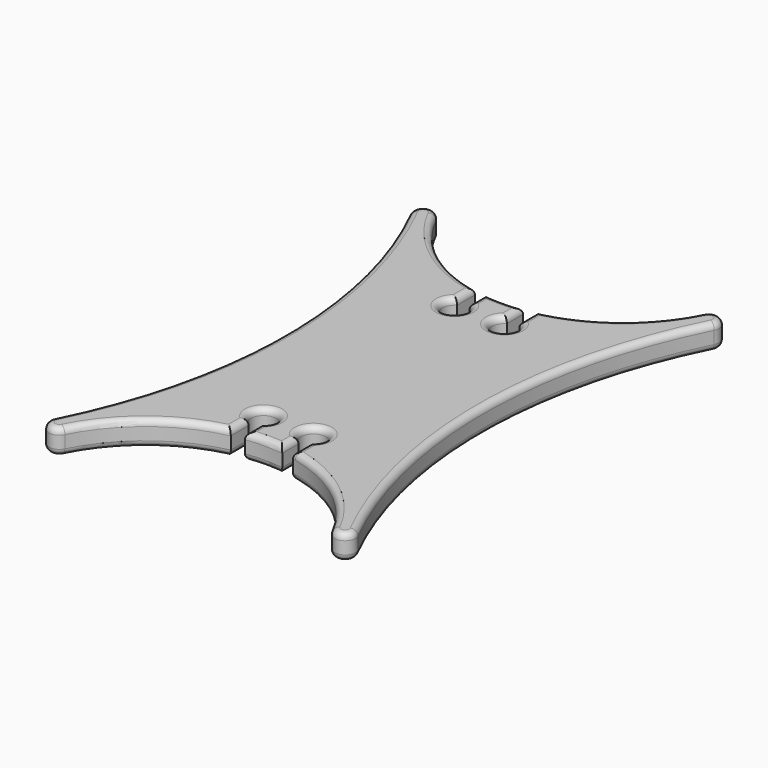
from build123d import *

# Parameters (mm, degrees)
F1_DEPTH     = 3.175
F2_T1_DEPTH  = 6.821932003
F2_T3_DEPTH  = 6.821932003
F2_T5_DEPTH  = 6.5533487431
F2_T7_DEPTH  = 6.5533487431
F2_T10_ANGLE = 359.64
F2_T12_ANGLE = 57.3793421658
F2_T14_ANGLE = 180
F2_T16_ANGLE = 53.1301023542
F2_T18_ANGLE = 180
F2_T20_ANGLE = 57.3793421658
F2_T22_ANGLE = 359.64
F2_T24_ANGLE = 26.298254359
F2_T26_ANGLE = 359.64
F2_T28_ANGLE = 57.3793421658
F2_T30_ANGLE = 180
F2_T32_ANGLE = 53.1301023542
F2_T34_ANGLE = 180
F2_T36_ANGLE = 57.3793421658
F2_T38_ANGLE = 359.64
F2_T40_ANGLE = 26.298254359
F2_T42_ANGLE = 359.64
F2_T44_ANGLE = 57.3793421658
F2_T46_ANGLE = 180
F2_T48_ANGLE = 53.1301023542
F2_T50_ANGLE = 180
F2_T52_ANGLE = 57.3793421658
F2_T54_ANGLE = 359.64
F2_T56_ANGLE = 26.298254359
F2_T58_ANGLE = 359.64
F2_T60_ANGLE = 57.3793421658
F2_T62_ANGLE = 180
F2_T64_ANGLE = 53.1301023542
F2_T66_ANGLE = 180
F2_T68_ANGLE = 57.3793421658
F2_T70_ANGLE = 359.64
F2_T72_ANGLE = 26.298254359


# Not quite as in the source:
# - a fillet or chamfer that OpenCascade refuses, or shapes differently, is made with other operations: its cross-section is extruded or revolved along the edge and cut away or added


with BuildPart() as f1:
    # F0 (on Top) → F1 (new body)
    with BuildSketch(Plane.XY):
        with BuildLine():
            ThreePointArc((-3.96875, 19.4679973315), (-11.6574343411, 23.0332576652), (-17.0388379885, 29.5805810057))
            ThreePointArc((-17.0388379885, 29.5805810057), (-18.8126145258, 30.1718398515), (-19.4038733715, 28.3980633142))
            ThreePointArc((-19.4038733715, 28.3980633142), (-12.7, 0), (-19.4038733715, -28.3980633142))
            ThreePointArc((-19.4038733715, -28.3980633142), (-18.8126145258, -30.1718398515), (-17.0388379885, -29.5805810057))
            ThreePointArc((-17.0388379885, -29.5805810057), (-11.6574343411, -23.0332576652), (-3.96875, -19.4679973315))
            Line((-3.96875, -19.4679973315), (-3.96875, -16.6148153285))
            ThreePointArc((-3.96875, -16.6148153285), (-3.175, -13.6525), (-2.38125, -16.6148153285))
            Line((-2.38125, -16.6148153285), (-2.38125, -19.1994140716))
            ThreePointArc((-2.38125, -19.1994140716), (0, -19.05), (2.38125, -19.1994140716))
            Line((2.38125, -19.1994140716), (2.38125, -16.6148153285))
            ThreePointArc((2.38125, -16.6148153285), (3.175, -13.6525), (3.96875, -16.6148153285))
            Line((3.96875, -16.6148153285), (3.96875, -19.4679973315))
            ThreePointArc((3.96875, -19.4679973315), (11.6574343411, -23.0332576652), (17.0388379885, -29.5805810057))
            ThreePointArc((17.0388379885, -29.5805810057), (18.8126145258, -30.1718398515), (19.4038733715, -28.3980633142))
            ThreePointArc((19.4038733715, -28.3980633142), (12.7, 0), (19.4038733715, 28.3980633142))
            ThreePointArc((19.4038733715, 28.3980633142), (18.8126145258, 30.1718398515), (17.0388379885, 29.5805810057))
            ThreePointArc((17.0388379885, 29.5805810057), (11.6574343411, 23.0332576652), (3.96875, 19.4679973315))
            Line((3.96875, 19.4679973315), (3.96875, 16.6148153285))
            ThreePointArc((3.96875, 16.6148153285), (3.175, 13.6525), (2.38125, 16.6148153285))
            Line((2.38125, 16.6148153285), (2.38125, 19.1994140716))
            ThreePointArc((2.38125, 19.1994140716), (0, 19.05), (-2.38125, 19.1994140716))
            Line((-2.38125, 19.1994140716), (-2.38125, 16.6148153285))
            ThreePointArc((-2.38125, 16.6148153285), (-3.175, 13.6525), (-3.96875, 16.6148153285))
            Line((-3.96875, 16.6148153285), (-3.96875, 19.4679973315))
        make_face()
    extrude(amount=F1_DEPTH)

    # F2: fillet of radius 0.79375 on 48 edges, made by hand

    # F2_s2 → F2_t1 (cut)
    with BuildSketch(Plane.XZ.offset(-21.4523723315)):
        with BuildLine():
            ThreePointArc((-3.96875, 2.38125), (-4.2012339924, 2.9425160076), (-4.7625, 3.175))
            Line((-4.7625, 3.175), (-3.96875, 3.175))
            Line((-3.96875, 3.175), (-3.96875, 2.38125))
        make_face()
        with BuildLine():
            ThreePointArc((3.96875, 2.38125), (4.2012339924, 2.9425160076), (4.7625, 3.175))
            Line((4.7625, 3.175), (3.96875, 3.175))
            Line((3.96875, 3.175), (3.96875, 2.38125))
        make_face()
        with BuildLine():
            ThreePointArc((-3.96875, 0.79375), (-4.2012339924, 0.2324839924), (-4.7625, 0))
            Line((-4.7625, 0), (-3.96875, 0))
            Line((-3.96875, 0), (-3.96875, 0.79375))
        make_face()
        with BuildLine():
            ThreePointArc((3.96875, 0.79375), (4.2012339924, 0.2324839924), (4.7625, 0))
            Line((4.7625, 0), (3.96875, 0))
            Line((3.96875, 0), (3.96875, 0.79375))
        make_face()
    extrude(amount=F2_T1_DEPTH, mode=Mode.SUBTRACT)

    # F2_s4 → F2_t3 (cut)
    with BuildSketch(Plane.XZ.offset(14.6304403285)):
        with BuildLine():
            ThreePointArc((-3.96875, 2.38125), (-4.2012339924, 2.9425160076), (-4.7625, 3.175))
            Line((-4.7625, 3.175), (-3.96875, 3.175))
            Line((-3.96875, 3.175), (-3.96875, 2.38125))
        make_face()
        with BuildLine():
            ThreePointArc((3.96875, 2.38125), (4.2012339924, 2.9425160076), (4.7625, 3.175))
            Line((4.7625, 3.175), (3.96875, 3.175))
            Line((3.96875, 3.175), (3.96875, 2.38125))
        make_face()
        with BuildLine():
            ThreePointArc((-3.96875, 0.79375), (-4.2012339924, 0.2324839924), (-4.7625, 0))
            Line((-4.7625, 0), (-3.96875, 0))
            Line((-3.96875, 0), (-3.96875, 0.79375))
        make_face()
        with BuildLine():
            ThreePointArc((3.96875, 0.79375), (4.2012339924, 0.2324839924), (4.7625, 0))
            Line((4.7625, 0), (3.96875, 0))
            Line((3.96875, 0), (3.96875, 0.79375))
        make_face()
    extrude(amount=F2_T3_DEPTH, mode=Mode.SUBTRACT)

    # F2_s6 → F2_t5 (cut)
    with BuildSketch(Plane.XZ.offset(14.6304403285)):
        with BuildLine():
            ThreePointArc((-2.38125, 2.38125), (-2.1487660076, 2.9425160076), (-1.5875, 3.175))
            Line((-1.5875, 3.175), (-2.38125, 3.175))
            Line((-2.38125, 3.175), (-2.38125, 2.38125))
        make_face()
        with BuildLine():
            ThreePointArc((2.38125, 2.38125), (2.1487660076, 2.9425160076), (1.5875, 3.175))
            Line((1.5875, 3.175), (2.38125, 3.175))
            Line((2.38125, 3.175), (2.38125, 2.38125))
        make_face()
        with BuildLine():
            ThreePointArc((-2.38125, 0.79375), (-2.1487660076, 0.2324839924), (-1.5875, 0))
            Line((-1.5875, 0), (-2.38125, 0))
            Line((-2.38125, 0), (-2.38125, 0.79375))
        make_face()
        with BuildLine():
            ThreePointArc((2.38125, 0.79375), (2.1487660076, 0.2324839924), (1.5875, 0))
            Line((1.5875, 0), (2.38125, 0))
            Line((2.38125, 0), (2.38125, 0.79375))
        make_face()
    extrude(amount=F2_T5_DEPTH, mode=Mode.SUBTRACT)

    # F2_s8 → F2_t7 (cut)
    with BuildSketch(Plane.XZ.offset(-21.1837890716)):
        with BuildLine():
            ThreePointArc((2.38125, 2.38125), (2.1487660076, 2.9425160076), (1.5875, 3.175))
            Line((1.5875, 3.175), (2.38125, 3.175))
            Line((2.38125, 3.175), (2.38125, 2.38125))
        make_face()
        with BuildLine():
            ThreePointArc((-2.38125, 2.38125), (-2.1487660076, 2.9425160076), (-1.5875, 3.175))
            Line((-1.5875, 3.175), (-2.38125, 3.175))
            Line((-2.38125, 3.175), (-2.38125, 2.38125))
        make_face()
        with BuildLine():
            ThreePointArc((2.38125, 0.79375), (2.1487660076, 0.2324839924), (1.5875, 0))
            Line((1.5875, 0), (2.38125, 0))
            Line((2.38125, 0), (2.38125, 0.79375))
        make_face()
        with BuildLine():
            ThreePointArc((-2.38125, 0.79375), (-2.1487660076, 0.2324839924), (-1.5875, 0))
            Line((-1.5875, 0), (-2.38125, 0))
            Line((-2.38125, 0), (-2.38125, 0.79375))
        make_face()
    extrude(amount=F2_T7_DEPTH, mode=Mode.SUBTRACT)

    # F2_s9 → F2_t10 (revolve, cut)
    with BuildSketch(Plane(origin=(-3.2228462211, 0.0101249033, 0), x_dir=(0, 0, 1), z_dir=(-0.9999950652, 0.0031415875, 0))):
        with BuildLine():
            ThreePointArc((2.38125, 16.8174502534), (2.9425160076, 17.0499342458), (3.175, 17.6112002534))
            Line((3.175, 17.6112002534), (3.175, 16.8174502534))
            Line((3.175, 16.8174502534), (2.38125, 16.8174502534))
        make_face()
    revolve(axis=Axis((-3.175, 15.24, 3.175), (0, 0, -1)), revolution_arc=F2_T10_ANGLE, mode=Mode.SUBTRACT)

    # F2_s11 → F2_t12 (revolve, cut)
    with BuildSketch(Plane(origin=(-3.9968789782, 0.4240112092, 0), x_dir=(0, 0, 1), z_dir=(0.9944199801, -0.1054936165, 0))):
        with BuildLine():
            ThreePointArc((2.38125, -18.8374012427), (2.9425160076, -18.6049172503), (3.175, -18.0436512427))
            Line((3.175, -18.0436512427), (3.175, -18.8374012427))
            Line((3.175, -18.8374012427), (2.38125, -18.8374012427))
        make_face()
    revolve(axis=Axis((0, 38.1, 3.175), (0, 0, -1)), revolution_arc=F2_T12_ANGLE, mode=Mode.SUBTRACT)

    # F2_s13 → F2_t14 (revolve, cut)
    with BuildSketch(Plane(origin=(-15.24, 30.48, 0), x_dir=(0, 0, 1), z_dir=(0.4472135955, -0.894427191, 0))):
        with BuildLine():
            ThreePointArc((2.38125, 2.0111620115), (2.9425160076, 2.2436460039), (3.175, 2.8049120115))
            Line((3.175, 2.8049120115), (3.175, 2.0111620115))
            Line((3.175, 2.0111620115), (2.38125, 2.0111620115))
        make_face()
    revolve(axis=Axis((-18.22135568, 28.98932216, 3.175), (0, 0, 1)), revolution_arc=F2_T14_ANGLE, mode=Mode.SUBTRACT)

    # F2_s15 → F2_t16 (revolve, cut)
    with BuildSketch(Plane(origin=(-15.24, 30.48, 0), x_dir=(0, 0, 1), z_dir=(-0.4472135955, 0.894427191, 0))):
        with BuildLine():
            ThreePointArc((2.38125, -4.6553519542), (2.9425160076, -4.4228679618), (3.175, -3.8616019542))
            Line((3.175, -3.8616019542), (3.175, -4.6553519542))
            Line((3.175, -4.6553519542), (2.38125, -4.6553519542))
        make_face()
    revolve(axis=Axis((-76.2, 0, 3.175), (0, 0, -1)), revolution_arc=F2_T16_ANGLE, mode=Mode.SUBTRACT)

    # F2_s17 → F2_t18 (revolve, cut)
    with BuildSketch(Plane(origin=(-15.24, -30.48, 0), x_dir=(0, 0, 1), z_dir=(0.4472135955, 0.894427191, 0))):
        with BuildLine():
            ThreePointArc((2.38125, -4.6553519542), (2.9425160076, -4.4228679618), (3.175, -3.8616019542))
            Line((3.175, -3.8616019542), (3.175, -4.6553519542))
            Line((3.175, -4.6553519542), (2.38125, -4.6553519542))
        make_face()
    revolve(axis=Axis((-18.22135568, -28.98932216, 3.175), (0, 0, 1)), revolution_arc=F2_T18_ANGLE, mode=Mode.SUBTRACT)

    # F2_s19 → F2_t20 (revolve, cut)
    with BuildSketch(Plane(origin=(-15.24, -30.48, 0), x_dir=(0, 0, 1), z_dir=(-0.4472135955, -0.894427191, 0))):
        with BuildLine():
            ThreePointArc((2.38125, 2.0111620115), (2.9425160076, 2.2436460039), (3.175, 2.8049120115))
            Line((3.175, 2.8049120115), (3.175, 2.0111620115))
            Line((3.175, 2.0111620115), (2.38125, 2.0111620115))
        make_face()
    revolve(axis=Axis((0, -38.1, 3.175), (0, 0, -1)), revolution_arc=F2_T20_ANGLE, mode=Mode.SUBTRACT)

    # F2_s21 → F2_t22 (revolve, cut)
    with BuildSketch(Plane(origin=(-3.1270911071, 0.0098240788, 0), x_dir=(0, 0, 1), z_dir=(0.9999950652, -0.0031415875, 0))):
        with BuildLine():
            ThreePointArc((2.38125, 16.8373993339), (2.9425160076, 17.0698833264), (3.175, 17.6311493339))
            Line((3.175, 17.6311493339), (3.175, 16.8373993339))
            Line((3.175, 16.8373993339), (2.38125, 16.8373993339))
        make_face()
    revolve(axis=Axis((-3.175, -15.24, 3.175), (0, 0, -1)), revolution_arc=F2_T22_ANGLE, mode=Mode.SUBTRACT)

    # F2_s23 → F2_t24 (revolve, cut)
    with BuildSketch(Plane(origin=(-8.4399858607, -1.9716763507, 0), x_dir=(0, 0, 1), z_dir=(-0.9737812714, -0.2274863412, 0))):
        with BuildLine():
            ThreePointArc((2.38125, -18.0510664407), (2.9425160076, -17.8185824483), (3.175, -17.2573164407))
            Line((3.175, -17.2573164407), (3.175, -18.0510664407))
            Line((3.175, -18.0510664407), (2.38125, -18.0510664407))
        make_face()
    revolve(axis=Axis((0, -38.1, 3.175), (0, 0, -1)), revolution_arc=F2_T24_ANGLE, mode=Mode.SUBTRACT)

    # F2_s25 → F2_t26 (revolve, cut)
    with BuildSketch(Plane(origin=(3.2228462211, -0.0101249033, 0), x_dir=(0, 0, 1), z_dir=(0.9999950652, -0.0031415875, 0))):
        with BuildLine():
            ThreePointArc((2.38125, 16.8174502534), (2.9425160076, 17.0499342458), (3.175, 17.6112002534))
            Line((3.175, 17.6112002534), (3.175, 16.8174502534))
            Line((3.175, 16.8174502534), (2.38125, 16.8174502534))
        make_face()
    revolve(axis=Axis((3.175, -15.24, 3.175), (0, 0, -1)), revolution_arc=F2_T26_ANGLE, mode=Mode.SUBTRACT)

    # F2_s27 → F2_t28 (revolve, cut)
    with BuildSketch(Plane(origin=(3.9968789782, -0.4240112092, 0), x_dir=(0, 0, 1), z_dir=(-0.9944199801, 0.1054936165, 0))):
        with BuildLine():
            ThreePointArc((2.38125, -18.8374012427), (2.9425160076, -18.6049172503), (3.175, -18.0436512427))
            Line((3.175, -18.0436512427), (3.175, -18.8374012427))
            Line((3.175, -18.8374012427), (2.38125, -18.8374012427))
        make_face()
    revolve(axis=Axis((0, -38.1, 3.175), (0, 0, -1)), revolution_arc=F2_T28_ANGLE, mode=Mode.SUBTRACT)

    # F2_s29 → F2_t30 (revolve, cut)
    with BuildSketch(Plane(origin=(15.24, -30.48, 0), x_dir=(0, 0, 1), z_dir=(-0.4472135955, 0.894427191, 0))):
        with BuildLine():
            ThreePointArc((2.38125, 2.0111620115), (2.9425160076, 2.2436460039), (3.175, 2.8049120115))
            Line((3.175, 2.8049120115), (3.175, 2.0111620115))
            Line((3.175, 2.0111620115), (2.38125, 2.0111620115))
        make_face()
    revolve(axis=Axis((18.22135568, -28.98932216, 3.175), (0, 0, 1)), revolution_arc=F2_T30_ANGLE, mode=Mode.SUBTRACT)

    # F2_s31 → F2_t32 (revolve, cut)
    with BuildSketch(Plane(origin=(15.24, -30.48, 0), x_dir=(0, 0, 1), z_dir=(0.4472135955, -0.894427191, 0))):
        with BuildLine():
            ThreePointArc((2.38125, -4.6553519542), (2.9425160076, -4.4228679618), (3.175, -3.8616019542))
            Line((3.175, -3.8616019542), (3.175, -4.6553519542))
            Line((3.175, -4.6553519542), (2.38125, -4.6553519542))
        make_face()
    revolve(axis=Axis((76.2, 0, 3.175), (0, 0, -1)), revolution_arc=F2_T32_ANGLE, mode=Mode.SUBTRACT)

    # F2_s33 → F2_t34 (revolve, cut)
    with BuildSketch(Plane(origin=(15.24, 30.48, 0), x_dir=(0, 0, 1), z_dir=(-0.4472135955, -0.894427191, 0))):
        with BuildLine():
            ThreePointArc((2.38125, -4.6553519542), (2.9425160076, -4.4228679618), (3.175, -3.8616019542))
            Line((3.175, -3.8616019542), (3.175, -4.6553519542))
            Line((3.175, -4.6553519542), (2.38125, -4.6553519542))
        make_face()
    revolve(axis=Axis((18.22135568, 28.98932216, 3.175), (0, 0, 1)), revolution_arc=F2_T34_ANGLE, mode=Mode.SUBTRACT)

    # F2_s35 → F2_t36 (revolve, cut)
    with BuildSketch(Plane(origin=(15.24, 30.48, 0), x_dir=(0, 0, 1), z_dir=(0.4472135955, 0.894427191, 0))):
        with BuildLine():
            ThreePointArc((2.38125, 2.0111620115), (2.9425160076, 2.2436460039), (3.175, 2.8049120115))
            Line((3.175, 2.8049120115), (3.175, 2.0111620115))
            Line((3.175, 2.0111620115), (2.38125, 2.0111620115))
        make_face()
    revolve(axis=Axis((0, 38.1, 3.175), (0, 0, -1)), revolution_arc=F2_T36_ANGLE, mode=Mode.SUBTRACT)

    # F2_s37 → F2_t38 (revolve, cut)
    with BuildSketch(Plane(origin=(3.1270911071, -0.0098240788, 0), x_dir=(0, 0, 1), z_dir=(-0.9999950652, 0.0031415875, 0))):
        with BuildLine():
            ThreePointArc((2.38125, 16.8373993339), (2.9425160076, 17.0698833264), (3.175, 17.6311493339))
            Line((3.175, 17.6311493339), (3.175, 16.8373993339))
            Line((3.175, 16.8373993339), (2.38125, 16.8373993339))
        make_face()
    revolve(axis=Axis((3.175, 15.24, 3.175), (0, 0, -1)), revolution_arc=F2_T38_ANGLE, mode=Mode.SUBTRACT)

    # F2_s39 → F2_t40 (revolve, cut)
    with BuildSketch(Plane(origin=(8.4399858607, 1.9716763507, 0), x_dir=(0, 0, 1), z_dir=(0.9737812714, 0.2274863412, 0))):
        with BuildLine():
            ThreePointArc((2.38125, -18.0510664407), (2.9425160076, -17.8185824483), (3.175, -17.2573164407))
            Line((3.175, -17.2573164407), (3.175, -18.0510664407))
            Line((3.175, -18.0510664407), (2.38125, -18.0510664407))
        make_face()
    revolve(axis=Axis((0, 38.1, 3.175), (0, 0, -1)), revolution_arc=F2_T40_ANGLE, mode=Mode.SUBTRACT)

    # F2_s41 → F2_t42 (revolve, cut)
    with BuildSketch(Plane(origin=(-3.2228462211, 0.0101249033, 0), x_dir=(0, 0, 1), z_dir=(-0.9999950652, 0.0031415875, 0))):
        with BuildLine():
            ThreePointArc((0.79375, 16.8174502534), (0.2324839924, 17.0499342458), (0, 17.6112002534))
            Line((0, 17.6112002534), (0, 16.8174502534))
            Line((0, 16.8174502534), (0.79375, 16.8174502534))
        make_face()
    revolve(axis=Axis((-3.175, 15.24, 0), (0, 0, -1)), revolution_arc=F2_T42_ANGLE, mode=Mode.SUBTRACT)

    # F2_s43 → F2_t44 (revolve, cut)
    with BuildSketch(Plane(origin=(-3.9968789782, 0.4240112092, 0), x_dir=(0, 0, 1), z_dir=(0.9944199801, -0.1054936165, 0))):
        with BuildLine():
            ThreePointArc((0.79375, -18.8374012427), (0.2324839924, -18.6049172503), (0, -18.0436512427))
            Line((0, -18.0436512427), (0, -18.8374012427))
            Line((0, -18.8374012427), (0.79375, -18.8374012427))
        make_face()
    revolve(axis=Axis((0, 38.1, 0), (0, 0, -1)), revolution_arc=F2_T44_ANGLE, mode=Mode.SUBTRACT)

    # F2_s45 → F2_t46 (revolve, cut)
    with BuildSketch(Plane(origin=(-15.24, 30.48, 0), x_dir=(0, 0, 1), z_dir=(0.4472135955, -0.894427191, 0))):
        with BuildLine():
            ThreePointArc((0.79375, 2.0111620115), (0.2324839924, 2.2436460039), (0, 2.8049120115))
            Line((0, 2.8049120115), (0, 2.0111620115))
            Line((0, 2.0111620115), (0.79375, 2.0111620115))
        make_face()
    revolve(axis=Axis((-18.22135568, 28.98932216, 0), (0, 0, 1)), revolution_arc=F2_T46_ANGLE, mode=Mode.SUBTRACT)

    # F2_s47 → F2_t48 (revolve, cut)
    with BuildSketch(Plane(origin=(-15.24, 30.48, 0), x_dir=(0, 0, 1), z_dir=(-0.4472135955, 0.894427191, 0))):
        with BuildLine():
            ThreePointArc((0.79375, -4.6553519542), (0.2324839924, -4.4228679618), (0, -3.8616019542))
            Line((0, -3.8616019542), (0, -4.6553519542))
            Line((0, -4.6553519542), (0.79375, -4.6553519542))
        make_face()
    revolve(axis=Axis((-76.2, 0, 0), (0, 0, -1)), revolution_arc=F2_T48_ANGLE, mode=Mode.SUBTRACT)

    # F2_s49 → F2_t50 (revolve, cut)
    with BuildSketch(Plane(origin=(-15.24, -30.48, 0), x_dir=(0, 0, 1), z_dir=(0.4472135955, 0.894427191, 0))):
        with BuildLine():
            ThreePointArc((0.79375, -4.6553519542), (0.2324839924, -4.4228679618), (0, -3.8616019542))
            Line((0, -3.8616019542), (0, -4.6553519542))
            Line((0, -4.6553519542), (0.79375, -4.6553519542))
        make_face()
    revolve(axis=Axis((-18.22135568, -28.98932216, 0), (0, 0, 1)), revolution_arc=F2_T50_ANGLE, mode=Mode.SUBTRACT)

    # F2_s51 → F2_t52 (revolve, cut)
    with BuildSketch(Plane(origin=(-15.24, -30.48, 0), x_dir=(0, 0, 1), z_dir=(-0.4472135955, -0.894427191, 0))):
        with BuildLine():
            ThreePointArc((0.79375, 2.0111620115), (0.2324839924, 2.2436460039), (0, 2.8049120115))
            Line((0, 2.8049120115), (0, 2.0111620115))
            Line((0, 2.0111620115), (0.79375, 2.0111620115))
        make_face()
    revolve(axis=Axis((0, -38.1, 0), (0, 0, -1)), revolution_arc=F2_T52_ANGLE, mode=Mode.SUBTRACT)

    # F2_s53 → F2_t54 (revolve, cut)
    with BuildSketch(Plane(origin=(-3.1270911071, 0.0098240788, 0), x_dir=(0, 0, 1), z_dir=(0.9999950652, -0.0031415875, 0))):
        with BuildLine():
            ThreePointArc((0.79375, 16.8373993339), (0.2324839924, 17.0698833264), (0, 17.6311493339))
            Line((0, 17.6311493339), (0, 16.8373993339))
            Line((0, 16.8373993339), (0.79375, 16.8373993339))
        make_face()
    revolve(axis=Axis((-3.175, -15.24, 0), (0, 0, -1)), revolution_arc=F2_T54_ANGLE, mode=Mode.SUBTRACT)

    # F2_s55 → F2_t56 (revolve, cut)
    with BuildSketch(Plane(origin=(-8.4399858607, -1.9716763507, 0), x_dir=(0, 0, 1), z_dir=(-0.9737812714, -0.2274863412, 0))):
        with BuildLine():
            ThreePointArc((0.79375, -18.0510664407), (0.2324839924, -17.8185824483), (0, -17.2573164407))
            Line((0, -17.2573164407), (0, -18.0510664407))
            Line((0, -18.0510664407), (0.79375, -18.0510664407))
        make_face()
    revolve(axis=Axis((0, -38.1, 0), (0, 0, -1)), revolution_arc=F2_T56_ANGLE, mode=Mode.SUBTRACT)

    # F2_s57 → F2_t58 (revolve, cut)
    with BuildSketch(Plane(origin=(3.2228462211, -0.0101249033, 0), x_dir=(0, 0, 1), z_dir=(0.9999950652, -0.0031415875, 0))):
        with BuildLine():
            ThreePointArc((0.79375, 16.8174502534), (0.2324839924, 17.0499342458), (0, 17.6112002534))
            Line((0, 17.6112002534), (0, 16.8174502534))
            Line((0, 16.8174502534), (0.79375, 16.8174502534))
        make_face()
    revolve(axis=Axis((3.175, -15.24, 0), (0, 0, -1)), revolution_arc=F2_T58_ANGLE, mode=Mode.SUBTRACT)

    # F2_s59 → F2_t60 (revolve, cut)
    with BuildSketch(Plane(origin=(3.9968789782, -0.4240112092, 0), x_dir=(0, 0, 1), z_dir=(-0.9944199801, 0.1054936165, 0))):
        with BuildLine():
            ThreePointArc((0.79375, -18.8374012427), (0.2324839924, -18.6049172503), (0, -18.0436512427))
            Line((0, -18.0436512427), (0, -18.8374012427))
            Line((0, -18.8374012427), (0.79375, -18.8374012427))
        make_face()
    revolve(axis=Axis((0, -38.1, 0), (0, 0, -1)), revolution_arc=F2_T60_ANGLE, mode=Mode.SUBTRACT)

    # F2_s61 → F2_t62 (revolve, cut)
    with BuildSketch(Plane(origin=(15.24, -30.48, 0), x_dir=(0, 0, 1), z_dir=(-0.4472135955, 0.894427191, 0))):
        with BuildLine():
            ThreePointArc((0.79375, 2.0111620115), (0.2324839924, 2.2436460039), (0, 2.8049120115))
            Line((0, 2.8049120115), (0, 2.0111620115))
            Line((0, 2.0111620115), (0.79375, 2.0111620115))
        make_face()
    revolve(axis=Axis((18.22135568, -28.98932216, 0), (0, 0, 1)), revolution_arc=F2_T62_ANGLE, mode=Mode.SUBTRACT)

    # F2_s63 → F2_t64 (revolve, cut)
    with BuildSketch(Plane(origin=(15.24, -30.48, 0), x_dir=(0, 0, 1), z_dir=(0.4472135955, -0.894427191, 0))):
        with BuildLine():
            ThreePointArc((0.79375, -4.6553519542), (0.2324839924, -4.4228679618), (0, -3.8616019542))
            Line((0, -3.8616019542), (0, -4.6553519542))
            Line((0, -4.6553519542), (0.79375, -4.6553519542))
        make_face()
    revolve(axis=Axis((76.2, 0, 0), (0, 0, -1)), revolution_arc=F2_T64_ANGLE, mode=Mode.SUBTRACT)

    # F2_s65 → F2_t66 (revolve, cut)
    with BuildSketch(Plane(origin=(15.24, 30.48, 0), x_dir=(0, 0, 1), z_dir=(-0.4472135955, -0.894427191, 0))):
        with BuildLine():
            ThreePointArc((0.79375, -4.6553519542), (0.2324839924, -4.4228679618), (0, -3.8616019542))
            Line((0, -3.8616019542), (0, -4.6553519542))
            Line((0, -4.6553519542), (0.79375, -4.6553519542))
        make_face()
    revolve(axis=Axis((18.22135568, 28.98932216, 0), (0, 0, 1)), revolution_arc=F2_T66_ANGLE, mode=Mode.SUBTRACT)

    # F2_s67 → F2_t68 (revolve, cut)
    with BuildSketch(Plane(origin=(15.24, 30.48, 0), x_dir=(0, 0, 1), z_dir=(0.4472135955, 0.894427191, 0))):
        with BuildLine():
            ThreePointArc((0.79375, 2.0111620115), (0.2324839924, 2.2436460039), (0, 2.8049120115))
            Line((0, 2.8049120115), (0, 2.0111620115))
            Line((0, 2.0111620115), (0.79375, 2.0111620115))
        make_face()
    revolve(axis=Axis((0, 38.1, 0), (0, 0, -1)), revolution_arc=F2_T68_ANGLE, mode=Mode.SUBTRACT)

    # F2_s69 → F2_t70 (revolve, cut)
    with BuildSketch(Plane(origin=(3.1270911071, -0.0098240788, 0), x_dir=(0, 0, 1), z_dir=(-0.9999950652, 0.0031415875, 0))):
        with BuildLine():
            ThreePointArc((0.79375, 16.8373993339), (0.2324839924, 17.0698833264), (0, 17.6311493339))
            Line((0, 17.6311493339), (0, 16.8373993339))
            Line((0, 16.8373993339), (0.79375, 16.8373993339))
        make_face()
    revolve(axis=Axis((3.175, 15.24, 0), (0, 0, -1)), revolution_arc=F2_T70_ANGLE, mode=Mode.SUBTRACT)

    # F2_s71 → F2_t72 (revolve, cut)
    with BuildSketch(Plane(origin=(8.4399858607, 1.9716763507, 0), x_dir=(0, 0, 1), z_dir=(0.9737812714, 0.2274863412, 0))):
        with BuildLine():
            ThreePointArc((0.79375, -18.0510664407), (0.2324839924, -17.8185824483), (0, -17.2573164407))
            Line((0, -17.2573164407), (0, -18.0510664407))
            Line((0, -18.0510664407), (0.79375, -18.0510664407))
        make_face()
    revolve(axis=Axis((0, 38.1, 0), (0, 0, -1)), revolution_arc=F2_T72_ANGLE, mode=Mode.SUBTRACT)


solid = f1.part
